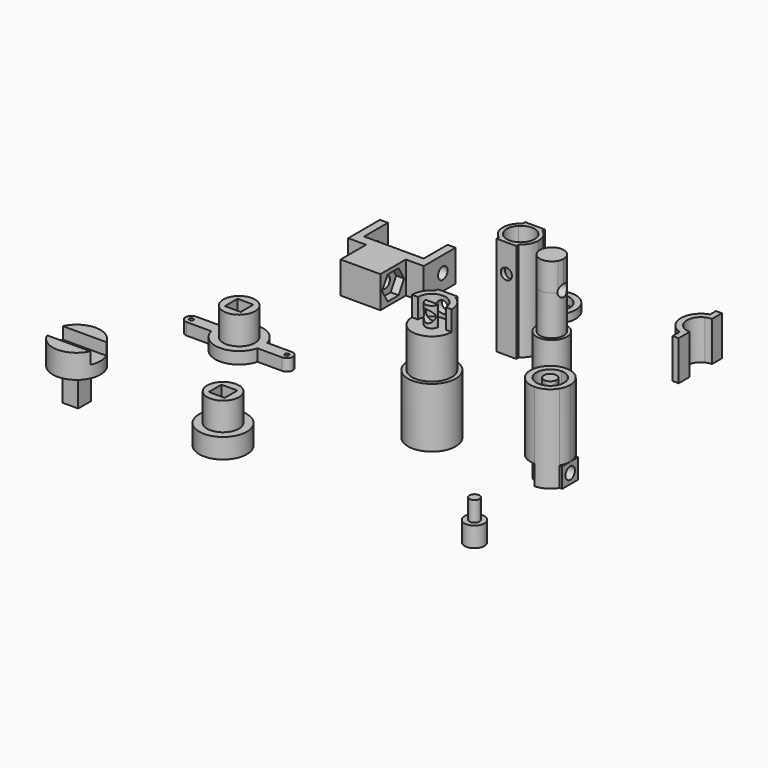
from build123d import *

# Parameters (mm, degrees)
F0_W      = 10
F0_H      = 8
F0_W_2    = 2
F0_H_2    = 7.5
F1_DEPTH  = 8
F2_R      = 1.5
F3_DEPTH  = 25
F4_R      = 1.5
F5_DEPTH  = 25
F7_DEPTH  = 15
F8_DEPTH  = 22
F9_DEPTH  = 5
F10_DEPTH = 5
F11_R     = 1.5
F12_DEPTH = 25
F13_R     = 6
F13_R_2   = 5
F13_R_3   = 3.9
F14_DEPTH = 15
F15_DEPTH = 10
F16_R     = 5
F17_DEPTH = 10
F19_DEPTH = 5
F20_R     = 1.5
F21_DEPTH = 25
F22_R     = 0.5
F23_DEPTH = 3
F24_R     = 4
F24_W     = 4
F24_H     = 4
F25_DEPTH = 7
F26_W     = 4
F26_H     = 4
F27_DEPTH = 8
F28_R     = 6
F28_W     = 2
F28_H     = 2
F29_DEPTH = 6
F31_DEPTH = 3
F32_R     = 6
F33_DEPTH = 5
F34_R     = 4
F34_W     = 4
F34_H     = 4
F35_DEPTH = 7
F37_DEPTH = 10
F39_DEPTH = 25
F38_R     = 1.55
F40_DEPTH = 4
F41_R     = 1.4
F42_DEPTH = 8
F43_R     = 3.8
F44_DEPTH = 10
F45_R     = 5
F45_R_2   = 3.5
F46_DEPTH = 2
F47_R     = 3
F48_DEPTH = 10
F50_DEPTH = 7
F52_R     = 1.5
F53_DEPTH = 6
F54_R     = 2.5
F54_R_2   = 1.25
F55_DEPTH = 5
F56_DEPTH = 10
F57_R     = 1.5
F58_DEPTH = 2
F59_R     = 1.5
F60_DEPTH = 2


with BuildPart() as f1:
    # F0 (on Top) → F1 (new body)
    with BuildSketch(Plane.XY):
        Polygon((-43.9805059528, 20.7387872934), (-39.4805059528, 20.7387872934), (-29.4805059528, 20.7387872934), (-24.9805059528, 20.7387872934), (-24.9805059528, 23.2387872934), (-26.9805059528, 23.2387872934), (-41.9805059528, 23.2387872934), (-43.9805059528, 23.2387872934), align=None)
        with Locations((-34.4805059528, 16.7387872934)):
            Rectangle(F0_W, F0_H)
        with Locations((-42.9805059528, 26.9887872934)):
            Rectangle(F0_W_2, F0_H_2)
        with Locations((-25.9805059528, 26.9887872934)):
            Rectangle(F0_W_2, F0_H_2)
    extrude(amount=F1_DEPTH)

    # F2 (on face) → F3 (cut)
    with BuildSketch(Plane(origin=(-39.4805059528, 0, 0), x_dir=(0, -1, 0), z_dir=(-1, 0, 0))):
        with Locations((-16.7387872934, 4)):
            Circle(F2_R)
    extrude(amount=-F3_DEPTH, mode=Mode.SUBTRACT)

    # F4 (on face) → F5 (cut)
    with BuildSketch(Plane(origin=(-43.9805059528, 0, 0), x_dir=(0, -1, 0), z_dir=(-1, 0, 0))):
        with Locations((-26.7387872934, 4)):
            Circle(F4_R)
    extrude(amount=-F5_DEPTH, mode=Mode.SUBTRACT)

    # F57 (on face) → F58 (cut)
    with BuildSketch(Plane(origin=(-39.4805059528, 0, 0), x_dir=(0, -1, 0), z_dir=(-1, 0, 0))):
        Polygon((-18.470838101, 1), (-15.0067364859, 1), (-13.2746856783, 4), (-15.0067364859, 7), (-18.470838101, 7), (-20.2028889086, 4), align=None)
        with Locations((-16.7387872934, 4)):
            Circle(F57_R, mode=Mode.SUBTRACT)
    extrude(amount=-F58_DEPTH, mode=Mode.SUBTRACT)

    # F59 (on face) → F60 (cut)
    with BuildSketch(Plane.YZ.offset(-29.4805059528)):
        Polygon((15.0067364859, 1), (18.470838101, 1), (20.2028889086, 4), (18.470838101, 7), (15.0067364859, 7), (13.2746856783, 4), align=None)
        with Locations((16.7387872934, 4)):
            Circle(F59_R, mode=Mode.SUBTRACT)
    extrude(amount=-F60_DEPTH, mode=Mode.SUBTRACT)


with BuildPart() as f7:
    # F6 (on Top) → F7 (new body)
    with BuildSketch(Plane.XY):
        with BuildLine():
            Line((40.8568046987, -20.1631552368), (40.8568046987, -18.2631552368))
            ThreePointArc((40.8568046987, -18.2631552368), (37.3568046987, -21.7631552368), (40.8568046987, -25.2631552368))
            Line((40.8568046987, -25.2631552368), (40.8568046987, -23.3631552368))
            ThreePointArc((40.8568046987, -23.3631552368), (39.2568046987, -21.7631552368), (40.8568046987, -20.1631552368))
        make_face()
        with BuildLine():
            ThreePointArc((44.3568046987, -21.7631552368), (43.3316784329, -19.2882815027), (40.8568046987, -18.2631552368))
            Line((40.8568046987, -18.2631552368), (40.8568046987, -20.1631552368))
            ThreePointArc((40.8568046987, -20.1631552368), (41.9881755486, -20.6317843869), (42.4568046987, -21.7631552368))
            ThreePointArc((42.4568046987, -21.7631552368), (41.9881755486, -22.8945260867), (40.8568046987, -23.3631552368))
            Line((40.8568046987, -23.3631552368), (40.8568046987, -25.2631552368))
            ThreePointArc((40.8568046987, -25.2631552368), (43.3316784329, -24.238028971), (44.3568046987, -21.7631552368))
        make_face()
    extrude(amount=F7_DEPTH)

    # F6 (on Top) → F8 (join)
    with BuildSketch(Plane.XY):
        with BuildLine():
            ThreePointArc((45.1869317176, -24.2631552368), (45.6864338302, -23.0572504624), (45.8568046987, -21.7631552368))
            ThreePointArc((45.8568046987, -21.7631552368), (45.6864338302, -20.4690600113), (45.1869317176, -19.2631552368))
            ThreePointArc((45.1869317176, -19.2631552368), (43.3568046987, -17.4330282179), (40.8568046987, -16.7631552368))
            Line((40.8568046987, -16.7631552368), (40.8568046987, -18.2631552368))
            ThreePointArc((40.8568046987, -18.2631552368), (43.3316784329, -19.2882815027), (44.3568046987, -21.7631552368))
            ThreePointArc((44.3568046987, -21.7631552368), (43.3316784329, -24.238028971), (40.8568046987, -25.2631552368))
            Line((40.8568046987, -25.2631552368), (40.8568046987, -26.7631552368))
            ThreePointArc((40.8568046987, -26.7631552368), (43.3568046987, -26.0932822558), (45.1869317176, -24.2631552368))
        make_face()
        with BuildLine():
            Line((40.8568046987, -23.3631552368), (40.8568046987, -20.1631552368))
            ThreePointArc((40.8568046987, -20.1631552368), (39.2568046987, -21.7631552368), (40.8568046987, -23.3631552368))
        make_face()
        with BuildLine():
            ThreePointArc((42.4568046987, -21.7631552368), (41.9881755486, -20.6317843869), (40.8568046987, -20.1631552368))
            Line((40.8568046987, -20.1631552368), (40.8568046987, -23.3631552368))
            ThreePointArc((40.8568046987, -23.3631552368), (41.9881755486, -22.8945260867), (42.4568046987, -21.7631552368))
        make_face()
        with BuildLine():
            Line((40.8568046987, -18.2631552368), (40.8568046987, -16.7631552368))
            ThreePointArc((40.8568046987, -16.7631552368), (35.8568046987, -21.7631552368), (40.8568046987, -26.7631552368))
            Line((40.8568046987, -26.7631552368), (40.8568046987, -25.2631552368))
            ThreePointArc((40.8568046987, -25.2631552368), (37.3568046987, -21.7631552368), (40.8568046987, -18.2631552368))
        make_face()
    extrude(amount=F8_DEPTH)

    # F6 (on Top) → F9 (cut)
    with BuildSketch(Plane.XY):
        with BuildLine():
            Line((40.8568046987, -18.2631552368), (40.8568046987, -16.7631552368))
            ThreePointArc((40.8568046987, -16.7631552368), (35.8568046987, -21.7631552368), (40.8568046987, -26.7631552368))
            Line((40.8568046987, -26.7631552368), (40.8568046987, -25.2631552368))
            ThreePointArc((40.8568046987, -25.2631552368), (37.3568046987, -21.7631552368), (40.8568046987, -18.2631552368))
        make_face()
        with BuildLine():
            ThreePointArc((42.4568046987, -21.7631552368), (41.9881755486, -20.6317843869), (40.8568046987, -20.1631552368))
            Line((40.8568046987, -20.1631552368), (40.8568046987, -23.3631552368))
            ThreePointArc((40.8568046987, -23.3631552368), (41.9881755486, -22.8945260867), (42.4568046987, -21.7631552368))
        make_face()
    extrude(amount=F9_DEPTH, mode=Mode.SUBTRACT)

    # F6 (on Top) → F10 (join)
    with BuildSketch(Plane.XY):
        with BuildLine():
            Line((45.8568046987, -24.2631552368), (45.8568046987, -21.7631552368))
            ThreePointArc((45.8568046987, -21.7631552368), (45.6864338302, -23.0572504624), (45.1869317176, -24.2631552368))
            Line((45.1869317176, -24.2631552368), (45.8568046987, -24.2631552368))
        make_face()
        with BuildLine():
            ThreePointArc((45.1869317176, -19.2631552368), (45.6864338302, -20.4690600113), (45.8568046987, -21.7631552368))
            Line((45.8568046987, -21.7631552368), (45.8568046987, -19.2631552368))
            Line((45.8568046987, -19.2631552368), (45.1869317176, -19.2631552368))
        make_face()
    extrude(amount=F10_DEPTH)

    # F11 (on face) → F12 (cut)
    with BuildSketch(Plane.YZ.offset(45.8568046987)):
        with Locations((-21.7631552368, 2.5)):
            Circle(F11_R)
    extrude(amount=-F12_DEPTH, mode=Mode.SUBTRACT)


with BuildPart() as f14:
    # F13 (on Top) → F14 (new body)
    with BuildSketch(Plane.XY):
        with Locations((12.2351311147, -23.2184566557)):
            Circle(F13_R)
        with Locations((12.2351311147, -23.2184566557)):
            Circle(F13_R_2, mode=Mode.SUBTRACT)
        with Locations((12.2351311147, -23.2184566557)):
            Circle(F13_R_2)
        with Locations((12.2351311147, -23.2184566557)):
            Circle(F13_R_3, mode=Mode.SUBTRACT)
        with Locations((12.2351311147, -23.2184566557)):
            Circle(F13_R_3)
    extrude(amount=F14_DEPTH)

    # F13 (on Top) → F15 (cut)
    with BuildSketch(Plane.XY):
        with Locations((12.2351311147, -23.2184566557)):
            Circle(F13_R_2)
        with Locations((12.2351311147, -23.2184566557)):
            Circle(F13_R_3, mode=Mode.SUBTRACT)
    extrude(amount=F15_DEPTH, mode=Mode.SUBTRACT)

    # F16 (on face) → F17 (join)
    with BuildSketch(Plane.XY.offset(15)):
        with Locations((12.2351311147, -23.2184566557)):
            Circle(F16_R)
    extrude(amount=F17_DEPTH)

    # F18 (on face) → F19 (join)
    with BuildSketch(Plane.XY.offset(25)):
        with BuildLine():
            Line((13.8351311147, -23.2184566557), (12.2351311147, -23.2184566557))
            Line((12.2351311147, -23.2184566557), (10.6351311147, -23.2184566557))
            ThreePointArc((10.6351311147, -23.2184566557), (12.2351311147, -24.8184566557), (13.8351311147, -23.2184566557))
        make_face()
        with BuildLine():
            Line((7.2351311147, -23.2184566557), (8.7351311147, -23.2184566557))
            ThreePointArc((8.7351311147, -23.2184566557), (12.2351311147, -19.7184566557), (15.7351311147, -23.2184566557))
            Line((15.7351311147, -23.2184566557), (17.2351311147, -23.2184566557))
            ThreePointArc((17.2351311147, -23.2184566557), (16.5652581336, -20.7184566557), (14.7351311147, -18.8883296368))
            ThreePointArc((14.7351311147, -18.8883296368), (13.5292263402, -18.3888275243), (12.2351311147, -18.2184566557))
            ThreePointArc((12.2351311147, -18.2184566557), (10.9410358892, -18.3888275243), (9.7351311147, -18.8883296368))
            ThreePointArc((9.7351311147, -18.8883296368), (7.9050040958, -20.7184566557), (7.2351311147, -23.2184566557))
        make_face()
        with BuildLine():
            Line((9.7351311147, -18.2184566557), (9.7351311147, -18.8883296368))
            ThreePointArc((9.7351311147, -18.8883296368), (10.9410358892, -18.3888275243), (12.2351311147, -18.2184566557))
            Line((12.2351311147, -18.2184566557), (9.7351311147, -18.2184566557))
        make_face()
        with BuildLine():
            ThreePointArc((12.2351311147, -18.2184566557), (13.5292263402, -18.3888275243), (14.7351311147, -18.8883296368))
            Line((14.7351311147, -18.8883296368), (14.7351311147, -18.2184566557))
            Line((14.7351311147, -18.2184566557), (12.2351311147, -18.2184566557))
        make_face()
    extrude(amount=F19_DEPTH)

    # F20 (on face) → F21 (cut)
    with BuildSketch(Plane(origin=(0, -18.2184566557, 0), x_dir=(-1, 0, 0), z_dir=(0, 1, 0))):
        with Locations((-12.2351311147, 27.5)):
            Circle(F20_R)
    extrude(amount=-F21_DEPTH, mode=Mode.SUBTRACT)


with BuildPart() as f23:
    # F22 (on Top) → F23 (new body)
    with BuildSketch(Plane.XY):
        with BuildLine():
            ThreePointArc((-52.4472220203, -19.447989516), (-51.3865618485, -19.0086496877), (-50.9472220203, -17.947989516))
            ThreePointArc((-50.9472220203, -17.947989516), (-51.3865618485, -16.8873293442), (-52.4472220203, -16.447989516))
            ThreePointArc((-52.4472220203, -16.447989516), (-53.9472220203, -17.947989516), (-52.4472220203, -19.447989516))
        make_face()
        with Locations((-52.4472220203, -17.947989516)):
            Circle(F22_R, mode=Mode.SUBTRACT)
        with BuildLine():
            ThreePointArc((-52.4472220203, -16.447989516), (-51.3865618485, -16.8873293442), (-50.9472220203, -17.947989516))
            Line((-50.9472220203, -17.947989516), (-46.4472220203, -17.947989516))
            ThreePointArc((-46.4472220203, -17.947989516), (-46.3994001979, -17.1919637611), (-46.2566970396, -16.447989516))
            Line((-46.2566970396, -16.447989516), (-52.4472220203, -16.447989516))
        make_face()
        with BuildLine():
            ThreePointArc((-46.2566970396, -16.447989516), (-46.3994001979, -17.1919637611), (-46.4472220203, -17.947989516))
            Line((-46.4472220203, -17.947989516), (-34.4472220203, -17.947989516))
            ThreePointArc((-34.4472220203, -17.947989516), (-34.4950438427, -17.1919637611), (-34.637747001, -16.447989516))
            Line((-34.637747001, -16.447989516), (-46.2566970396, -16.447989516))
        make_face()
        with BuildLine():
            ThreePointArc((-34.637747001, -16.447989516), (-34.4950438427, -17.1919637611), (-34.4472220203, -17.947989516))
            Line((-34.4472220203, -17.947989516), (-29.9472220203, -17.947989516))
            ThreePointArc((-29.9472220203, -17.947989516), (-29.5078821921, -16.8873293442), (-28.4472220203, -16.447989516))
            Line((-28.4472220203, -16.447989516), (-34.637747001, -16.447989516))
        make_face()
        with BuildLine():
            ThreePointArc((-28.4472220203, -16.447989516), (-29.5078821921, -16.8873293442), (-29.9472220203, -17.947989516))
            ThreePointArc((-29.9472220203, -17.947989516), (-29.5078821921, -19.0086496877), (-28.4472220203, -19.447989516))
            ThreePointArc((-28.4472220203, -19.447989516), (-27.3865618485, -19.0086496877), (-26.9472220203, -17.947989516))
            ThreePointArc((-26.9472220203, -17.947989516), (-27.3865618485, -16.8873293442), (-28.4472220203, -16.447989516))
        make_face()
        with BuildLine():
            ThreePointArc((-27.9472220203, -17.947989516), (-28.4472220203, -18.447989516), (-28.9472220203, -17.947989516))
            ThreePointArc((-28.9472220203, -17.947989516), (-28.4472220203, -17.447989516), (-27.9472220203, -17.947989516))
        make_face(mode=Mode.SUBTRACT)
        with BuildLine():
            Line((-46.4472220203, -17.947989516), (-50.9472220203, -17.947989516))
            ThreePointArc((-50.9472220203, -17.947989516), (-51.3865618485, -19.0086496877), (-52.4472220203, -19.447989516))
            Line((-52.4472220203, -19.447989516), (-46.2566970396, -19.447989516))
            ThreePointArc((-46.2566970396, -19.447989516), (-46.3994001979, -18.7040152709), (-46.4472220203, -17.947989516))
        make_face()
        with BuildLine():
            Line((-34.4472220203, -17.947989516), (-46.4472220203, -17.947989516))
            ThreePointArc((-46.4472220203, -17.947989516), (-46.3994001979, -18.7040152709), (-46.2566970396, -19.447989516))
            Line((-46.2566970396, -19.447989516), (-34.637747001, -19.447989516))
            ThreePointArc((-34.637747001, -19.447989516), (-34.4950438427, -18.7040152709), (-34.4472220203, -17.947989516))
        make_face()
        with BuildLine():
            Line((-34.637747001, -19.447989516), (-46.2566970396, -19.447989516))
            ThreePointArc((-46.2566970396, -19.447989516), (-40.4472220203, -23.947989516), (-34.637747001, -19.447989516))
        make_face()
        with BuildLine():
            Line((-29.9472220203, -17.947989516), (-34.4472220203, -17.947989516))
            ThreePointArc((-34.4472220203, -17.947989516), (-34.4950438427, -18.7040152709), (-34.637747001, -19.447989516))
            Line((-34.637747001, -19.447989516), (-28.4472220203, -19.447989516))
            ThreePointArc((-28.4472220203, -19.447989516), (-29.5078821921, -19.0086496877), (-29.9472220203, -17.947989516))
        make_face()
        with BuildLine():
            ThreePointArc((-34.637747001, -16.447989516), (-40.4472220203, -11.947989516), (-46.2566970396, -16.447989516))
            Line((-46.2566970396, -16.447989516), (-34.637747001, -16.447989516))
        make_face()
    extrude(amount=F23_DEPTH)

    # F24 (on face) → F25 (join)
    with BuildSketch(Plane.XY.offset(3)):
        with Locations((-40.4472220203, -17.947989516)):
            Circle(F24_R)
        with Locations((-40.4472220203, -17.947989516)):
            Rectangle(F24_W, F24_H, mode=Mode.SUBTRACT)
    extrude(amount=F25_DEPTH)


with BuildPart() as f27:
    # F26 (on Top) → F27 (new body)
    with BuildSketch(Plane.XY):
        with Locations((-51.7097190022, -54.951852884)):
            Rectangle(F26_W, F26_H)
    extrude(amount=F27_DEPTH)

    # F28 (on face) → F29 (join)
    with BuildSketch(Plane.XY.offset(8)):
        with Locations((-51.7097190022, -54.951852884)):
            Circle(F28_R)
        Polygon((-49.7097190022, -56.951852884), (-51.7097190022, -56.951852884), (-53.7097190022, -56.951852884), (-53.7097190022, -54.951852884), (-53.7097190022, -52.951852884), (-51.7097190022, -52.951852884), (-49.7097190022, -52.951852884), (-49.7097190022, -54.951852884), align=None, mode=Mode.SUBTRACT)
        with Locations((-52.7097190022, -55.951852884)):
            Rectangle(F28_W, F28_H)
        with Locations((-50.7097190022, -55.951852884)):
            Rectangle(F28_W, F28_H)
        with Locations((-50.7097190022, -53.951852884)):
            Rectangle(F28_W, F28_H)
        with Locations((-52.7097190022, -53.951852884)):
            Rectangle(F28_W, F28_H)
    extrude(amount=F29_DEPTH)

    # F30 (on face) → F31 (cut)
    with BuildSketch(Plane.XY.offset(14)):
        with BuildLine():
            ThreePointArc((-57.1640750596, -52.451852884), (-57.7097190022, -54.951852884), (-57.1640750596, -57.451852884))
            Line((-57.1640750596, -57.451852884), (-46.2553629449, -57.451852884))
            ThreePointArc((-46.2553629449, -57.451852884), (-45.8477169405, -56.2312792508), (-45.7097190022, -54.951852884))
            ThreePointArc((-45.7097190022, -54.951852884), (-45.8477169405, -53.6724265172), (-46.2553629449, -52.451852884))
            Line((-46.2553629449, -52.451852884), (-57.1640750596, -52.451852884))
        make_face()
    extrude(amount=-F31_DEPTH, mode=Mode.SUBTRACT)


with BuildPart() as f33:
    # F32 (on Top) → F33 (new body)
    with BuildSketch(Plane.XY):
        with Locations((-17.6909044385, -51.4450073242)):
            Circle(F32_R)
    extrude(amount=F33_DEPTH)

    # F34 (on face) → F35 (join)
    with BuildSketch(Plane.XY.offset(5)):
        with Locations((-17.6909044385, -51.4450073242)):
            Circle(F34_R)
        with Locations((-17.6909044385, -51.4450073242)):
            Rectangle(F34_W, F34_H, mode=Mode.SUBTRACT)
    extrude(amount=F35_DEPTH)


with BuildPart() as f37:
    # F36 (on Top) → F37 (new body)
    with BuildSketch(Plane.XY):
        with BuildLine():
            Line((35.6613672684, 25.0815060425), (35.6613672684, 27.035195309))
            ThreePointArc((35.6613672684, 27.035195309), (34.9025787719, 27.0931066799), (34.1613672684, 27.2654993019))
            Line((34.1613672684, 27.2654993019), (34.1613672684, 25.0815060425))
            Line((34.1613672684, 25.0815060425), (35.6613672684, 25.0815060425))
        make_face()
        with BuildLine():
            ThreePointArc((34.1613672684, 27.2654993019), (34.9025787719, 27.0931066799), (35.6613672684, 27.035195309))
            Line((35.6613672684, 27.035195309), (35.6613672684, 28.535195309))
            ThreePointArc((35.6613672684, 28.535195309), (34.8925928576, 28.6206695871), (34.1613672684, 28.8729176488))
            Line((34.1613672684, 28.8729176488), (34.1613672684, 27.2654993019))
        make_face()
        with BuildLine():
            Line((34.1613672684, 35.1974729692), (34.1613672684, 36.8048913161))
            ThreePointArc((34.1613672684, 36.8048913161), (30.6613672684, 32.035195309), (34.1613672684, 27.2654993019))
            Line((34.1613672684, 27.2654993019), (34.1613672684, 28.8729176488))
            ThreePointArc((34.1613672684, 28.8729176488), (32.1613672684, 32.035195309), (34.1613672684, 35.1974729692))
        make_face()
        with BuildLine():
            Line((35.6613672684, 35.535195309), (35.6613672684, 37.035195309))
            ThreePointArc((35.6613672684, 37.035195309), (34.9025787719, 36.9772839381), (34.1613672684, 36.8048913161))
            Line((34.1613672684, 36.8048913161), (34.1613672684, 35.1974729692))
            ThreePointArc((34.1613672684, 35.1974729692), (34.8925928576, 35.4497210309), (35.6613672684, 35.535195309))
        make_face()
        with BuildLine():
            ThreePointArc((34.1613672684, 36.8048913161), (34.9025787719, 36.9772839381), (35.6613672684, 37.035195309))
            Line((35.6613672684, 37.035195309), (35.6613672684, 38.6745472935))
            Line((35.6613672684, 38.6745472935), (34.1613672684, 38.6745472935))
            Line((34.1613672684, 38.6745472935), (34.1613672684, 36.8048913161))
        make_face()
    extrude(amount=F37_DEPTH)


with BuildPart() as f39:
    # F38 (on Top) → F39 (new body)
    with BuildSketch(Plane.XY):
        with BuildLine():
            Line((4.2699520662, 20.2254334393), (4.2699520662, 21.5176010833))
            ThreePointArc((4.2699520662, 21.5176010833), (3.0761951063, 22.0821867366), (1.7699520662, 22.2759436965))
            ThreePointArc((1.7699520662, 22.2759436965), (0.4637090262, 22.0821867366), (-0.7300479338, 21.5176010833))
            Line((-0.7300479338, 21.5176010833), (-0.7300479338, 20.2254334393))
            ThreePointArc((-0.7300479338, 20.2254334393), (1.7699520662, 21.2759436965), (4.2699520662, 20.2254334393))
        make_face()
        with BuildLine():
            ThreePointArc((1.7699520662, 13.2759436965), (3.0761951063, 13.4697006564), (4.2699520662, 14.0342863097))
            Line((4.2699520662, 14.0342863097), (4.2699520662, 15.3264539537))
            ThreePointArc((4.2699520662, 15.3264539537), (1.7699520662, 14.2759436965), (-0.7300479338, 15.3264539537))
            Line((-0.7300479338, 15.3264539537), (-0.7300479338, 14.0342863097))
            ThreePointArc((-0.7300479338, 14.0342863097), (0.4637090262, 13.4697006564), (1.7699520662, 13.2759436965))
        make_face()
        with BuildLine():
            ThreePointArc((4.2699520662, 14.0342863097), (5.7385790328, 15.6546233529), (6.2699520662, 17.7759436965))
            ThreePointArc((6.2699520662, 17.7759436965), (5.7385790328, 19.8972640401), (4.2699520662, 21.5176010833))
            Line((4.2699520662, 21.5176010833), (4.2699520662, 20.2254334393))
            ThreePointArc((4.2699520662, 20.2254334393), (5.0103224154, 19.098819352), (5.2699520662, 17.7759436965))
            ThreePointArc((5.2699520662, 17.7759436965), (5.0103224154, 16.453068041), (4.2699520662, 15.3264539537))
            Line((4.2699520662, 15.3264539537), (4.2699520662, 14.0342863097))
        make_face()
        with BuildLine():
            Line((-0.7300479338, 20.2254334393), (-0.7300479338, 21.5176010833))
            ThreePointArc((-0.7300479338, 21.5176010833), (-2.7300479338, 17.7759436965), (-0.7300479338, 14.0342863097))
            Line((-0.7300479338, 14.0342863097), (-0.7300479338, 15.3264539537))
            ThreePointArc((-0.7300479338, 15.3264539537), (-1.7300479338, 17.7759436965), (-0.7300479338, 20.2254334393))
        make_face()
        with BuildLine():
            Line((4.2699520662, 13.2759436965), (4.2699520662, 14.0342863097))
            ThreePointArc((4.2699520662, 14.0342863097), (3.0761951063, 13.4697006564), (1.7699520662, 13.2759436965))
            Line((1.7699520662, 13.2759436965), (4.2699520662, 13.2759436965))
        make_face()
        with BuildLine():
            ThreePointArc((1.7699520662, 22.2759436965), (3.0761951063, 22.0821867366), (4.2699520662, 21.5176010833))
            Line((4.2699520662, 21.5176010833), (4.2699520662, 22.2759436965))
            Line((4.2699520662, 22.2759436965), (1.7699520662, 22.2759436965))
        make_face()
        with BuildLine():
            ThreePointArc((-0.7300479338, 21.5176010833), (0.4637090262, 22.0821867366), (1.7699520662, 22.2759436965))
            Line((1.7699520662, 22.2759436965), (-0.7300479338, 22.2759436965))
            Line((-0.7300479338, 22.2759436965), (-0.7300479338, 21.5176010833))
        make_face()
        with BuildLine():
            Line((-0.7300479338, 13.2759436965), (1.7699520662, 13.2759436965))
            ThreePointArc((1.7699520662, 13.2759436965), (0.4637090262, 13.4697006564), (-0.7300479338, 14.0342863097))
            Line((-0.7300479338, 14.0342863097), (-0.7300479338, 13.2759436965))
        make_face()
    extrude(amount=F39_DEPTH)

    # F38 (on Top) → F40 (join)
    with BuildSketch(Plane.XY):
        with BuildLine():
            Line((4.2699520662, 15.3264539537), (4.2699520662, 20.2254334393))
            ThreePointArc((4.2699520662, 20.2254334393), (1.7699520662, 21.2759436965), (-0.7300479338, 20.2254334393))
            Line((-0.7300479338, 20.2254334393), (-0.7300479338, 15.3264539537))
            ThreePointArc((-0.7300479338, 15.3264539537), (1.7699520662, 14.2759436965), (4.2699520662, 15.3264539537))
        make_face()
        with Locations((1.7699520662, 17.7759436965)):
            Circle(F38_R, mode=Mode.SUBTRACT)
        with BuildLine():
            ThreePointArc((5.2699520662, 17.7759436965), (5.0103224154, 19.098819352), (4.2699520662, 20.2254334393))
            Line((4.2699520662, 20.2254334393), (4.2699520662, 15.3264539537))
            ThreePointArc((4.2699520662, 15.3264539537), (5.0103224154, 16.453068041), (5.2699520662, 17.7759436965))
        make_face()
        with BuildLine():
            Line((-0.7300479338, 15.3264539537), (-0.7300479338, 20.2254334393))
            ThreePointArc((-0.7300479338, 20.2254334393), (-1.7300479338, 17.7759436965), (-0.7300479338, 15.3264539537))
        make_face()
    extrude(amount=F40_DEPTH)

    # F41 (on face) → F42 (cut)
    with BuildSketch(Plane.XZ.offset(-13.2759436965)):
        with Locations((1.7699520662, 18)):
            Circle(F41_R)
    extrude(amount=-F42_DEPTH, mode=Mode.SUBTRACT)


with BuildPart() as f44:
    # F43 (on Top) → F44 (new body)
    with BuildSketch(Plane.XY):
        with Locations((14.3589694053, 11.8313347921)):
            Circle(F43_R)
    extrude(amount=F44_DEPTH)

    # F47 (on face) → F48 (join)
    with BuildSketch(Plane.XY.offset(10)):
        with Locations((14.3589694053, 11.8313347921)):
            Circle(F47_R)
    extrude(amount=F48_DEPTH)

    # F49 (on face) → F50 (join)
    with BuildSketch(Plane.XY.offset(20)):
        with BuildLine():
            ThreePointArc((17.0122692376, 10.4313347921), (17.2710047328, 11.1101896946), (17.3589694053, 11.8313347921))
            ThreePointArc((17.3589694053, 11.8313347921), (17.2710047328, 12.5524798895), (17.0122692376, 13.2313347921))
            Line((17.0122692376, 13.2313347921), (11.705669573, 13.2313347921))
            ThreePointArc((11.705669573, 13.2313347921), (11.4469340778, 12.5524798895), (11.3589694053, 11.8313347921))
            ThreePointArc((11.3589694053, 11.8313347921), (11.4469340778, 11.1101896946), (11.705669573, 10.4313347921))
            Line((11.705669573, 10.4313347921), (17.0122692376, 10.4313347921))
        make_face()
        with BuildLine():
            Line((11.705669573, 13.2313347921), (17.0122692376, 13.2313347921))
            ThreePointArc((17.0122692376, 13.2313347921), (14.3589694053, 14.8313347921), (11.705669573, 13.2313347921))
        make_face()
        with BuildLine():
            ThreePointArc((11.705669573, 10.4313347921), (14.3589694053, 8.8313347921), (17.0122692376, 10.4313347921))
            Line((17.0122692376, 10.4313347921), (11.705669573, 10.4313347921))
        make_face()
    extrude(amount=F50_DEPTH)

    # F52 (on line) → F53 (cut)
    with BuildSketch(Plane(origin=(17.3589694053, 0, 0), x_dir=(0, -1, 0), z_dir=(-1, 0, 0))):
        with Locations((-11.8311615661, 19.9998766184)):
            Circle(F52_R)
    extrude(amount=F53_DEPTH, mode=Mode.SUBTRACT)


with BuildPart() as f46:
    # F45 (on Top) → F46 (new body)
    with BuildSketch(Plane.XY):
        with Locations((-2.2269852925, 33.8337235153)):
            Circle(F45_R)
        with Locations((-2.2269852925, 33.8337235153)):
            Circle(F45_R_2, mode=Mode.SUBTRACT)
    extrude(amount=F46_DEPTH)


with BuildPart() as f55:
    # F54 (on Top) → F55 (new body)
    with BuildSketch(Plane.XY):
        with Locations((46.5924181044, -52.763313055)):
            Circle(F54_R)
        with Locations((46.5924181044, -52.763313055)):
            Circle(F54_R_2, mode=Mode.SUBTRACT)
    extrude(amount=F55_DEPTH)

    # F54 (on Top) → F56 (join)
    with BuildSketch(Plane.XY):
        with Locations((46.5924181044, -52.763313055)):
            Circle(F54_R_2)
    extrude(amount=F56_DEPTH)


solid = Compound([f1.part, f7.part, f14.part, f23.part, f27.part, f33.part, f37.part, f39.part, f44.part, f46.part, f55.part])
